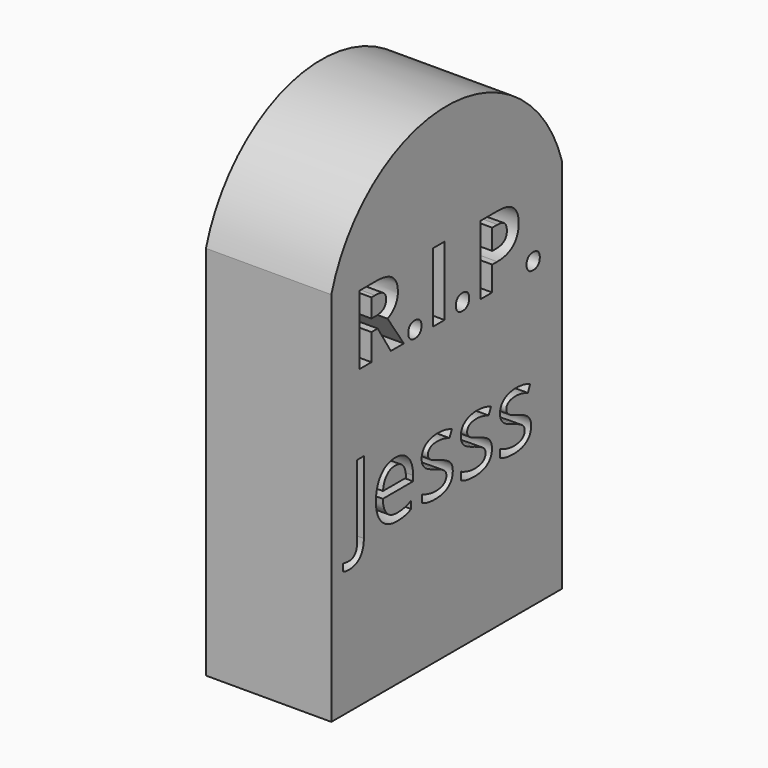
from build123d import *

# Parameters (mm, degrees)
F0_W         = 58.42
F0_H         = 76.2
F1_DEPTH     = 25.4
F2_DEPTH     = 25.4
F3_TEXT_SIZE = 20.7873889142
F4_DEPTH     = 15.24
F5_TEXT_SIZE = 19.5867821781
F6_DEPTH     = 15.24
F7_TEXT_SIZE = 5.2803765155
F8_DEPTH     = 25.4


# Not quite as in the source:
# - Text() gives the source's letters only with a copy of the font that has no kerning and outlines rounded to 1/6400 em; it was checked with that copy


with BuildPart() as f1:
    # F0 (on Right) → F1 (new body)
    with BuildSketch(Plane.YZ):
        with Locations((11.4057403614, -6.0917665079)):
            Rectangle(F0_W, F0_H)
    extrude(amount=F1_DEPTH)

    # F0 (on Right) → F2 (join)
    with BuildSketch(Plane.YZ):
        with Locations((11.4057403614, -6.0917665079)):
            Rectangle(F0_W, F0_H)
        with BuildLine():
            ThreePointArc((40.6157403614, 32.0082334921), (11.4057403614, 53.7815521495), (-17.8042596386, 32.0082334921))
            Line((-17.8042596386, 32.0082334921), (40.6157403614, 32.0082334921))
        make_face()
    extrude(amount=F2_DEPTH)

    # F3 (on face) → F4 (cut)
    with BuildSketch(Plane.YZ.offset(25.4)):
        with Locations((-13.2292363988, -14.9669200182)):
            Text('Jesss', F3_TEXT_SIZE, font='Open Sans', text_align=(TextAlign.LEFT, TextAlign.BOTTOM))
    extrude(amount=-F4_DEPTH, mode=Mode.SUBTRACT)

    # F5 (on face) → F6 (cut)
    with BuildSketch(Plane.YZ.offset(25.4)):
        with Locations((-12.3756458052, 15.8293154091)):
            Text('R.I.P.', F5_TEXT_SIZE, font='Open Sans', font_style=FontStyle.BOLD, text_align=(TextAlign.LEFT, TextAlign.BOTTOM))
    extrude(amount=-F6_DEPTH, mode=Mode.SUBTRACT)

    # F7 (on Right) → F8 (join)
    with BuildSketch(Plane.YZ):
        with Locations((-15.5167412013, -36.5263074636)):
            Text('2000-2016', F7_TEXT_SIZE, font='Open Sans', text_align=(TextAlign.LEFT, TextAlign.BOTTOM))
    extrude(amount=F8_DEPTH)


solid = f1.part
